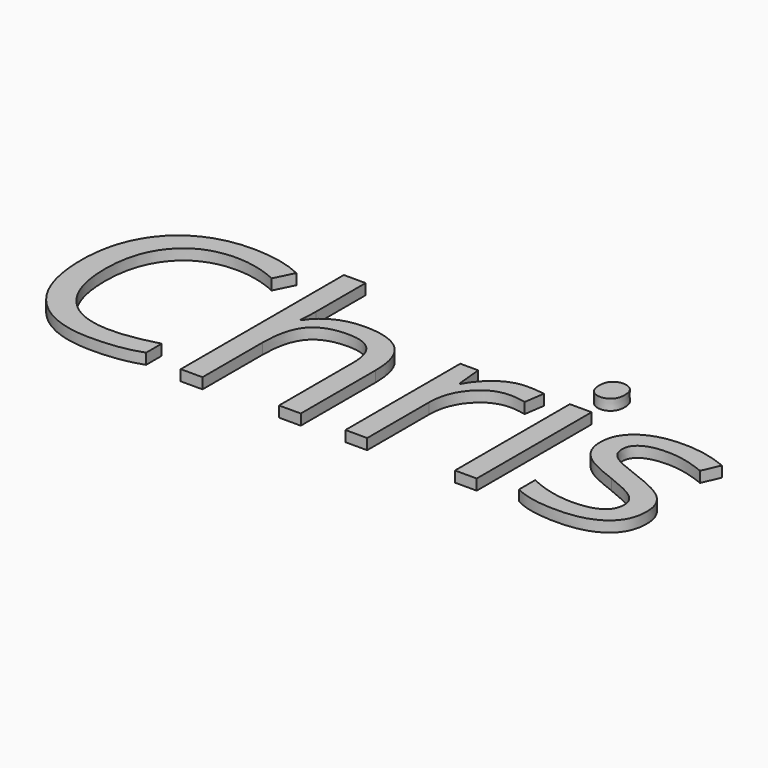
from build123d import *

# Parameters (mm, degrees)
F0_TEXT_SIZE = 31.725214676
F1_DEPTH     = 1.27


# Not quite as in the source:
# - Text() gives the source's letters only with a copy of the font that has no kerning and outlines rounded to 1/6400 em; it was checked with that copy


with BuildPart() as f1:
    # F0 (on Top) → F1 (new body)
    with BuildSketch(Plane.XY):
        with Locations((-20.6373237795, -16.2186915096)):
            Text('Chris', F0_TEXT_SIZE, font='Open Sans', text_align=(TextAlign.LEFT, TextAlign.BOTTOM))
    extrude(amount=F1_DEPTH)


solid = f1.part
